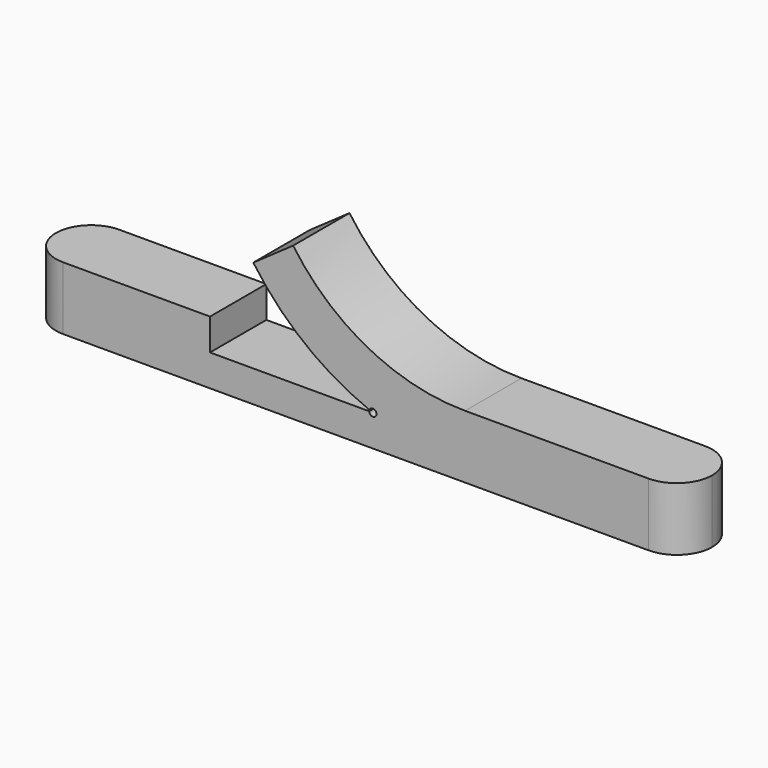
from build123d import *

# Parameters (mm, degrees)
F2_DEPTH = 2.9
F3_R     = 1.44999
F4_D     = 0.3


# Not quite as in the source:
# - a fillet or chamfer is up to 0.001 mm smaller than in the source, because OpenCascade refuses the exact size


with BuildPart() as f2:
    # F0 (on Front) → F2 (new body)
    with BuildSketch(Plane.XZ):
        Polygon((9.0052141035, -8.636), (0, -8.636), (0, -9.936), (-3.7947858965, -9.936), (-10.4947858965, -9.936), (-10.4947858965, -8.636), (-17.9947858965, -8.636), (-17.9947858965, -11.236), (9.0052141035, -11.236), align=None)
        with BuildLine():
            Line((0, -9.936), (0, -8.636))
            ThreePointArc((0, -8.636), (-3.9876610239, -7.6602255553), (-7.0741970545, -4.9534061043))
            Line((-7.0741970545, -4.9534061043), (-8.7125011431, -6.100558977))
            ThreePointArc((-8.7125011431, -6.100558977), (-6.5410785986, -8.3868222091), (-3.7947858965, -9.936))
            Line((-3.7947858965, -9.936), (0, -9.936))
        make_face()
    extrude(amount=F2_DEPTH)

    # F3 (radius 1.45 in the source; OpenCascade refuses exactly that, so slightly less here)
    f3_edges = [f2.edges().sort_by_distance(p)[0] for p in [
        (9.005214, -2.9, -9.936),
        (9.005214, 0, -9.936),
        (-17.994786, -2.9, -9.936),
        (-17.994786, 0, -9.936),
    ]]
    fillet(f3_edges, radius=F3_R)

    # F4 (through all)
    with Locations(Plane(origin=(0, 0, 0), x_dir=(1, 0, 0), z_dir=(0, 1, 0))):
        with Locations((-3.7947858965, 9.936)):
            Hole(F4_D / 2)


solid = f2.part
